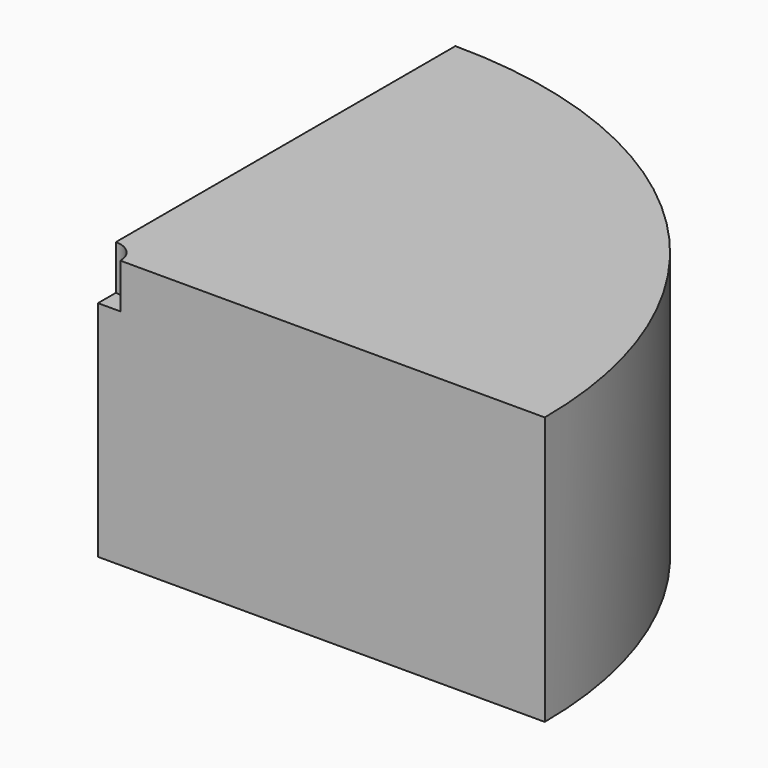
from build123d import *

# Parameters (mm, degrees)
F3_DEPTH = 6
F4_DEPTH = 1


# Not quite as in the source:
# - a feature of the source that left no trace in its solid (it failed there, or was rolled back) is left out


with BuildPart() as f3:
    # F0 (on Top) → F3 (new body)
    with BuildSketch(Plane.XY):
        with BuildLine():
            ThreePointArc((0, 1.25), (0.8838834765, 0.8838834765), (1.25, 0))
            Line((1.25, 0), (10, 0))
            ThreePointArc((10, 0), (7.0710678119, 7.0710678119), (0, 10))
            Line((0, 10), (0, 1.25))
        make_face()
        with BuildLine():
            ThreePointArc((0, 0.5), (0.3535533906, 0.3535533906), (0.5, 0))
            Line((0.5, 0), (1.25, 0))
            ThreePointArc((1.25, 0), (0.8838834765, 0.8838834765), (0, 1.25))
            Line((0, 1.25), (0, 0.5))
        make_face()
        with BuildLine():
            Line((0, 0), (0.5, 0))
            ThreePointArc((0.5, 0), (0.3535533906, 0.3535533906), (0, 0.5))
            Line((0, 0.5), (0, 0))
        make_face()
    extrude(amount=-F3_DEPTH)

    # F0 (on Top) → F4 (cut)
    with BuildSketch(Plane.XY):
        with BuildLine():
            Line((0, 0), (0.5, 0))
            ThreePointArc((0.5, 0), (0.3535533906, 0.3535533906), (0, 0.5))
            Line((0, 0.5), (0, 0))
        make_face()
    extrude(amount=-F4_DEPTH, mode=Mode.SUBTRACT)


solid = f3.part
